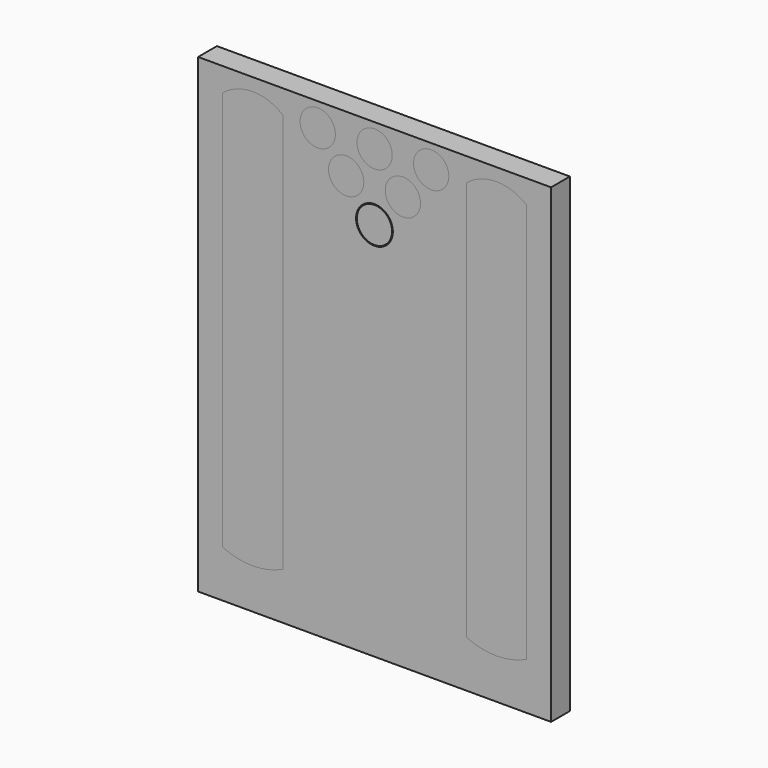
from build123d import *

# Parameters (mm, degrees)
F0_R     = 3.969461057
F0_R_2   = 3.81
F2_DEPTH = 5.08
F3_R     = 3.81
F4_DEPTH = 3.81


# Not quite as in the source:
# - the program builds the solid bodies; features that only make, move or delete a surface that nothing else refers to are left out


with BuildPart() as f2:
    # F0 (on Front) → F2 (new body)
    with BuildSketch(Plane.XZ):
        Polygon((34.9182439864, 43.0892817676), (-41.2817560136, 43.0892817676), (-41.2817560136, -58.5107182324), (34.9182439864, -58.5107182324), (34.9182439864, 38.0092817676), align=None)
        with BuildLine():
            ThreePointArc((-35.9619408846, 38.0092817676), (-29.4849408846, 40.3415061576), (-23.0079408846, 38.0092817676))
            Line((-23.0079408846, 38.0092817676), (-23.0079408846, -48.3507182324))
            ThreePointArc((-23.0079408846, -48.3507182324), (-29.4849408846, -49.7955715858), (-35.9619408846, -48.3507182324))
            Line((-35.9619408846, -48.3507182324), (-35.9619408846, 38.0092817676))
        make_face(mode=Mode.SUBTRACT)
        with Locations((-3.2106578548, 23.5410566752)):
            Circle(F0_R, mode=Mode.SUBTRACT)
        with BuildLine():
            ThreePointArc((-19.2659630901, 38.0092817676), (-15.4559630901, 41.8192817676), (-11.6459630901, 38.0092817676))
            ThreePointArc((-11.6459630901, 38.0092817676), (-15.4559630901, 34.1992817676), (-19.2659630901, 38.0092817676))
        make_face(mode=Mode.SUBTRACT)
        with Locations((-9.3160557696, 30.8942313745)):
            Circle(F0_R_2, mode=Mode.SUBTRACT)
        with BuildLine():
            ThreePointArc((16.6556439864, 38.0092817676), (23.1326439864, 40.3415061576), (29.6096439864, 38.0092817676))
            Line((29.6096439864, 38.0092817676), (29.6096439864, -48.3507182324))
            ThreePointArc((29.6096439864, -48.3507182324), (23.1326439864, -49.7955715858), (16.6556439864, -48.3507182324))
            Line((16.6556439864, -48.3507182324), (16.6556439864, 38.0092817676))
        make_face(mode=Mode.SUBTRACT)
        with Locations((2.9297477686, 30.8650228573)):
            Circle(F0_R_2, mode=Mode.SUBTRACT)
        with BuildLine():
            ThreePointArc((-6.9861484491, 38.0092817676), (-3.1761484491, 41.8192817676), (0.6338515509, 38.0092817676))
            ThreePointArc((0.6338515509, 38.0092817676), (-3.1761484491, 34.1992817676), (-6.9861484491, 38.0092817676))
        make_face(mode=Mode.SUBTRACT)
        with BuildLine():
            ThreePointArc((5.2256439864, 38.0092817676), (9.0356439864, 41.8192817676), (12.8456439864, 38.0092817676))
            ThreePointArc((12.8456439864, 38.0092817676), (9.0356439864, 34.1992817676), (5.2256439864, 38.0092817676))
        make_face(mode=Mode.SUBTRACT)
    extrude(amount=F2_DEPTH)


with BuildPart() as f4:
    # F3 (on face) → F4 (new body)
    with BuildSketch(Plane.XZ.offset(5.08)):
        with Locations((-15.4559630901, 38.0092817676)):
            Circle(F3_R)
    extrude(amount=-F4_DEPTH)


with BuildPart() as f4b:
    # F3 (on face) → F4, piece 2 (new body)
    with BuildSketch(Plane.XZ.offset(5.08)):
        with Locations((-3.1761484491, 38.0092817676)):
            Circle(F3_R)
    extrude(amount=-F4_DEPTH)


with BuildPart() as f4c:
    # F3 (on face) → F4, piece 3 (new body)
    with BuildSketch(Plane.XZ.offset(5.08)):
        with Locations((9.0356439864, 38.0092817676)):
            Circle(F3_R)
    extrude(amount=-F4_DEPTH)


with BuildPart() as f4d:
    # F3 (on face) → F4, piece 4 (new body)
    with BuildSketch(Plane.XZ.offset(5.08)):
        with Locations((2.9297477686, 30.8650228573)):
            Circle(F3_R)
    extrude(amount=-F4_DEPTH)


with BuildPart() as f4e:
    # F3 (on face) → F4, piece 5 (new body)
    with BuildSketch(Plane.XZ.offset(5.08)):
        with Locations((-9.3160557696, 30.8942313745)):
            Circle(F3_R)
    extrude(amount=-F4_DEPTH)


with BuildPart() as f4f:
    # F3 (on face) → F4, piece 6 (new body)
    with BuildSketch(Plane.XZ.offset(5.08)):
        with Locations((-3.2106578548, 23.5410566752)):
            Circle(F3_R)
    extrude(amount=-F4_DEPTH)


with BuildPart() as f4g:
    # F3 (on face) → F4, piece 7 (new body)
    with BuildSketch(Plane.XZ.offset(5.08)):
        with BuildLine():
            Line((-23.0079408846, -48.3507182324), (-23.0079408846, 38.0092817676))
            ThreePointArc((-23.0079408846, 38.0092817676), (-29.4849408846, 40.2938211878), (-35.9619408846, 38.0092817676))
            Line((-35.9619408846, 38.0092817676), (-35.9619408846, -48.3507182324))
            ThreePointArc((-35.9619408846, -48.3507182324), (-29.4849408846, -49.7955715858), (-23.0079408846, -48.3507182324))
        make_face()
        with BuildLine():
            ThreePointArc((-35.9619408846, 38.0092817676), (-29.4849408846, 40.2938211878), (-23.0079408846, 38.0092817676))
            ThreePointArc((-23.0079408846, 38.0092817676), (-29.4849408846, 40.3415061576), (-35.9619408846, 38.0092817676))
        make_face()
    extrude(amount=-F4_DEPTH)


with BuildPart() as f4h:
    # F3 (on face) → F4, piece 8 (new body)
    with BuildSketch(Plane.XZ.offset(5.08)):
        with BuildLine():
            Line((29.6096439864, -48.3507182324), (29.6096439864, 38.0092817676))
            ThreePointArc((29.6096439864, 38.0092817676), (23.1326439864, 40.3415061576), (16.6556439864, 38.0092817676))
            Line((16.6556439864, 38.0092817676), (16.6556439864, -48.3507182324))
            ThreePointArc((16.6556439864, -48.3507182324), (23.1326439864, -49.7955715858), (29.6096439864, -48.3507182324))
        make_face()
    extrude(amount=-F4_DEPTH)


solid = Compound([f2.part, f4.part, f4b.part, f4c.part, f4d.part, f4e.part, f4f.part, f4g.part, f4h.part])
